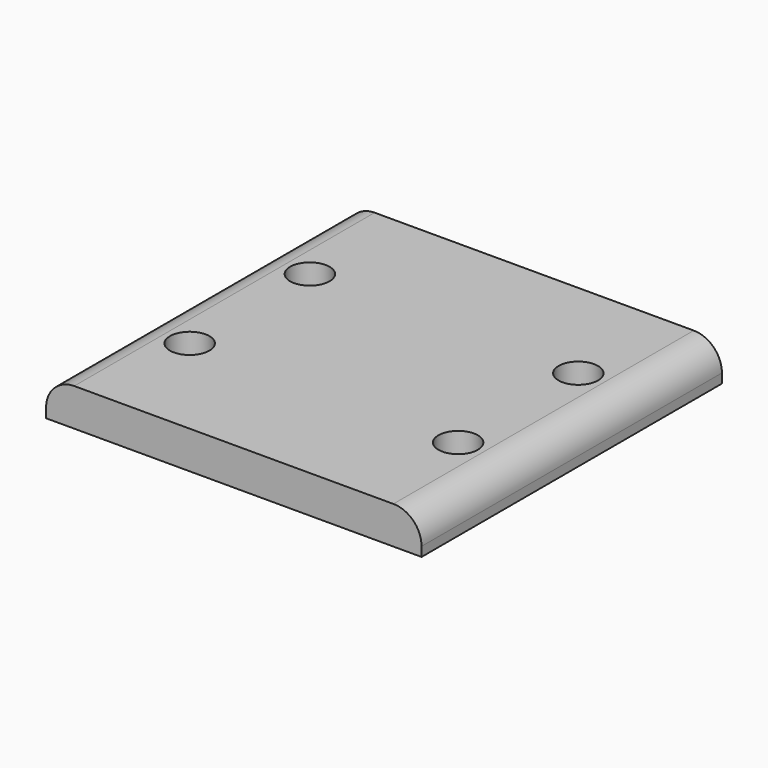
from build123d import *

# Parameters (mm, degrees)
F0_W     = 40
F0_H     = 40
F1_DEPTH = 8
F2_R     = 2.1
F3_DEPTH = 25
F4_W     = 40
F4_H     = 4
F5_DEPTH = 100
F6_R     = 3


# Not quite as in the source:
# - a feature names something its author has since deleted; it is built from what else it names


with BuildPart() as f1:
    # F0 (on Top) → F1 (new body)
    with BuildSketch(Plane.XY):
        with Locations((20, 20)):
            Rectangle(F0_W, F0_H)
    extrude(amount=F1_DEPTH)

    # F2 (on face) → F3 (cut)
    with BuildSketch(Plane.XY.offset(8)):
        with Locations((5.7, 12)):
            Circle(F2_R)
        with Locations((5.7, 28)):
            Circle(F2_R)
        with Locations((34.3, 28)):
            Circle(F2_R)
        with Locations((34.3, 12)):
            Circle(F2_R)
    extrude(amount=-F3_DEPTH, mode=Mode.SUBTRACT)

    # F4 (on face) → F5 (cut)
    with BuildSketch(Plane(origin=(0, 40, 0), x_dir=(-1, 0, 0), z_dir=(0, 1, 0))):
        with Locations((-20, 6)):
            Rectangle(F4_W, F4_H)
    extrude(amount=-F5_DEPTH, mode=Mode.SUBTRACT)

    # F6
    f6_edges = [f1.edges().sort_by_distance(p)[0] for p in [
        (0, 20, 4),
        (40, 20, 4),
    ]]
    fillet(f6_edges, radius=F6_R)


solid = f1.part
